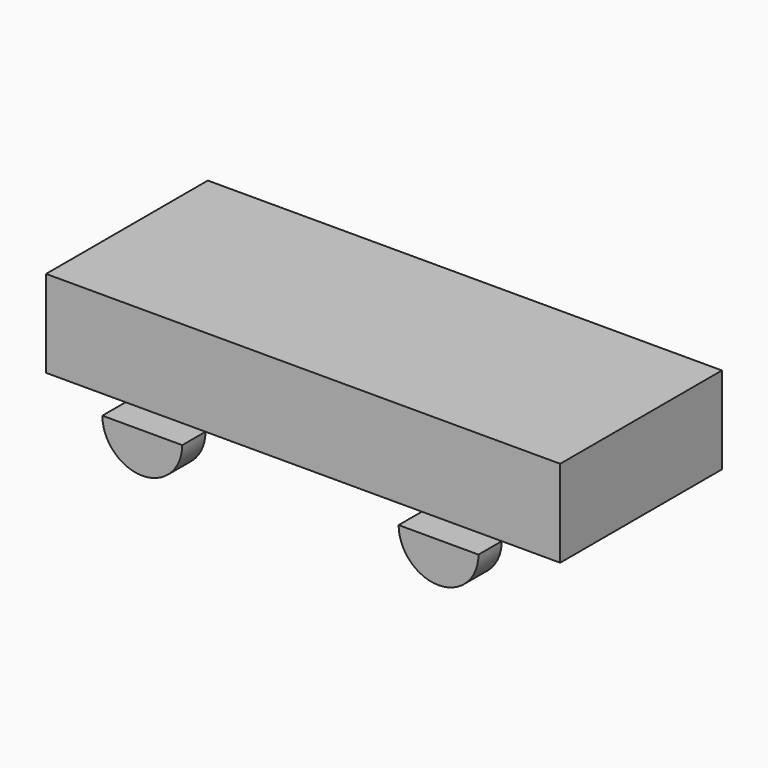
from build123d import *

# Parameters (mm, degrees)
F0_W     = 449.58
F0_H     = 176.784
F1_DEPTH = 76.2
F3_DEPTH = 25.4


with BuildPart() as f1:
    # F0 (on Top) → F1 (new body)
    with BuildSketch(Plane.XY):
        with Locations((98.376634287, 0.3670174628)):
            Rectangle(F0_W, F0_H)
    extrude(amount=F1_DEPTH)


with BuildPart() as f3:
    # F2 (on face) → F3 (new body)
    with BuildSketch(Plane.XZ.offset(88.0249825372)):
        with BuildLine():
            ThreePointArc((-56.8707894564, 0), (-21.9457894564, -34.925), (12.9792105436, 0))
            Line((12.9792105436, 0), (-56.8707894564, 0))
        make_face()
    extrude(amount=F3_DEPTH)


with BuildPart() as f3b:
    # F2 (on face) → F3, piece 2 (new body)
    with BuildSketch(Plane.XZ.offset(88.0249825372)):
        with BuildLine():
            Line((272.0592105436, 0), (202.2092105436, 0))
            ThreePointArc((202.2092105436, 0), (237.1342105436, -34.925), (272.0592105436, 0))
        make_face()
    extrude(amount=F3_DEPTH)


solid = Compound([f1.part, f3.part, f3b.part])
